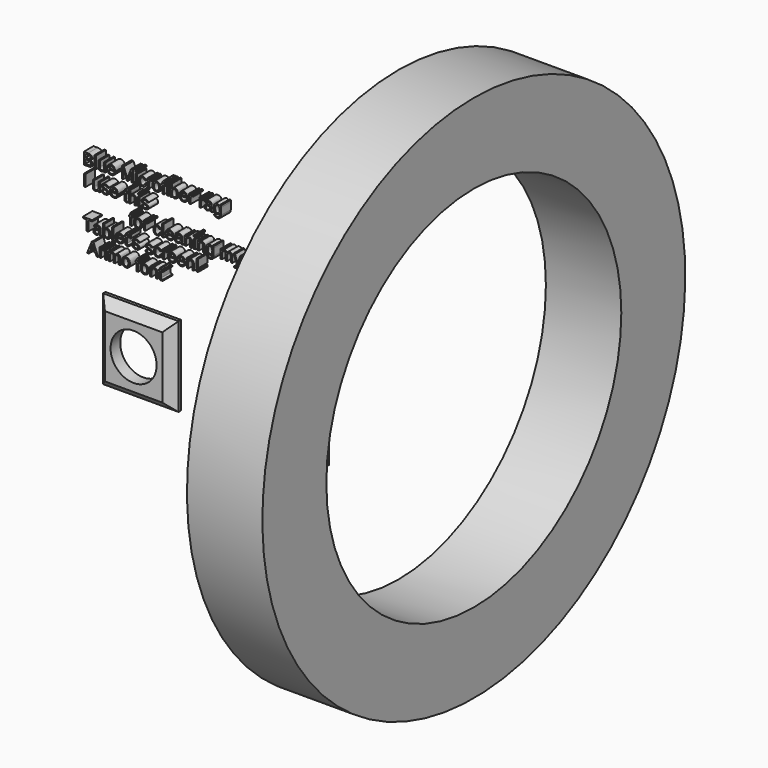
from build123d import *

# Parameters (mm, degrees)
F4_W         = 158.75
F4_H         = 168.275
F4_TEXT_SIZE = 35.0679167443
F5_DEPTH     = 25.4
F0_W         = 158.75
F0_H         = 168.275
F1_DEPTH     = 0.5953125
F6_SIZE      = 19.05
F2_R         = 48.4839772265
F7_DEPTH     = 25.4
F3_W         = 158.75
F3_H         = 168.275


# Not quite as in the source:
# - a length typed as a fraction of an inch, garbled in the dataset ("3 / 203.2 mm" for 3/8 in), is restored
# - Text() gives the source's letters only with a copy of the font that has no kerning and outlines rounded to 1/6400 em; it was checked with that copy


with BuildPart() as f5:
    # F4 (on Front) → F5 (new body)
    with BuildSketch(Plane.XZ):
        with Locations((79.375, 84.1375)):
            Rectangle(F4_W, F4_H)
        with Locations((-28.3411368728, 406.0246795416)):
            Text('Blue Microfiber rag', F4_TEXT_SIZE, font='Arimo', text_align=(TextAlign.LEFT, TextAlign.BOTTOM))
        with Locations((-28.3411368728, 365.6965752857)):
            Text('I use this', F4_TEXT_SIZE, font='Arimo', text_align=(TextAlign.LEFT, TextAlign.BOTTOM))
        with Locations((69.0819193324, 325.3684710297)):
            Text('for cleaning my', F4_TEXT_SIZE, font='Arimo', text_align=(TextAlign.LEFT, TextAlign.BOTTOM))
        with Locations((-28.3411368728, 285.0403667738)):
            Text("Tablet's screen!", F4_TEXT_SIZE, font='Arimo', text_align=(TextAlign.LEFT, TextAlign.BOTTOM))
        with Locations((-18.5988312522, 244.7122625179)):
            Text('Arimo font', F4_TEXT_SIZE, font='Arimo', text_align=(TextAlign.LEFT, TextAlign.BOTTOM))
    extrude(amount=F5_DEPTH)

    # F6
    f6_edges = [f5.edges().sort_by_distance(p)[0] for p in [
        (158.75, -25.4, 84.1375),
        (79.375, -25.4, 0),
        (0, -25.4, 84.1375),
        (79.375, -25.4, 168.275),
    ]]
    chamfer(f6_edges, length=F6_SIZE)

    # F2 (on face) → F7 (cut)
    with BuildSketch(Plane.XZ.offset(25.4)):
        with Locations((79.375, 84.1375)):
            Circle(F2_R)
    extrude(amount=-F7_DEPTH, mode=Mode.SUBTRACT)


with BuildPart() as f1:
    # F0 (on Front) → F1 (new body)
    with BuildSketch(Plane.XZ):
        with Locations((391.2116412646, 84.1375)):
            Rectangle(F0_W, F0_H)
    extrude(amount=F1_DEPTH)


with BuildPart() as f8:
    # F3 (on Front) → F8 (revolve)
    with BuildSketch(Plane.XZ):
        with Locations((695.7191824913, 695.9125379332)):
            Rectangle(F3_W, F3_H)
    revolve(axis=Axis((722.9421138763, 0, 223.7702906132), (1, 0, 0)))


solid = Compound([f5.part, f1.part, f8.part])
